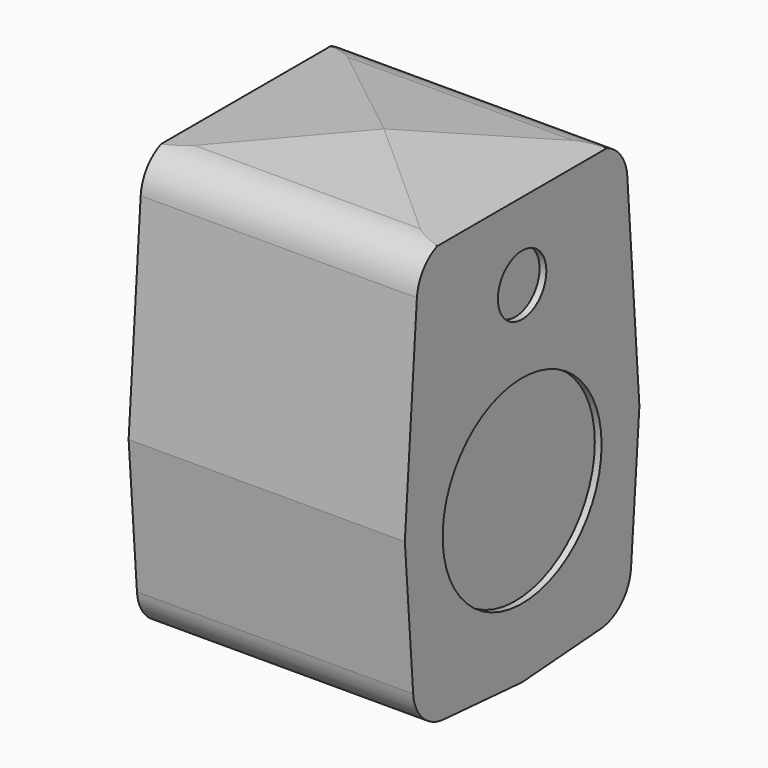
from build123d import *

# Parameters (mm, degrees)
F0_W         = 121
F0_H         = 195
F1_DEPTH     = 114
F3_DEPTH     = 114
F4_R         = 17
F6_DEPTH     = 134.1
F7_DEPTH     = 135.6
F2_R         = 41
F2_R_2       = 12.5
F8_DEPTH     = 2.8
F9_W         = 71.5012215078
F9_H         = 111.9857653975
F10_DEPTH    = 5
F11_W        = 35
F11_H        = 35
F12_DEPTH    = 35
F13_R        = 15
F14_DEPTH    = 35
F15_T1_DEPTH = 123.1187950266


# Not quite as in the source:
# - a fillet or chamfer that OpenCascade refuses, or shapes differently, is made with other operations: its cross-section is extruded or revolved along the edge and cut away or added


with BuildPart() as f1:
    # F0 (on Right) → F1 (new body)
    with BuildSketch(Plane.YZ):
        with Locations((-7.0141647011, 35.3717551942)):
            Rectangle(F0_W, F0_H)
    extrude(amount=F1_DEPTH)

    # F2 (on face) → F3 (cut, through all)
    with BuildSketch(Plane.YZ.offset(114)):
        Polygon((-60.2907269257, 126.0077205761), (-7.0141647011, 132.8717551942), (-67.5141647011, 132.8717551942), (-67.5141647011, 26.0932128876), align=None)
        Polygon((53.4858352989, 132.8717551942), (-7.0141647011, 132.8717551942), (46.2623975235, 126.0077205761), (53.4858352989, 26.0932128876), align=None)
        Polygon((-62.1019659576, -45.638720619), (-67.5141647011, 26.0932128876), (-67.5141647011, -62.1282448058), (53.4858352989, -62.1282448058), (53.4858352989, 26.0932128876), (48.0736365554, -45.638720619), (-7.0141647011, -49.6213585138), align=None)
    extrude(amount=-F3_DEPTH, mode=Mode.SUBTRACT)

    # F4
    f4_edges = [f1.edges().sort_by_distance(p)[0] for p in [
        (57, -60.290727, 126.007721),
        (57, 46.262398, 126.007721),
        (57, 48.073637, -45.638721),
        (57, -62.101966, -45.638721),
    ]]
    fillet(f4_edges, radius=F4_R)

    # F5 (on Front) → F6 (cut)
    with BuildSketch(Plane.XZ):
        Polygon((56.9999999998, 132.8717551942), (-2e-10, 132.8717551942), (-2e-10, 126.6480237246), align=None)
        Polygon((113.9999999999, 132.8717551942), (56.9999999998, 132.8717551942), (113.9999999999, 126.6480237246), align=None)
    extrude(amount=-F6_DEPTH, mode=Mode.SUBTRACT)

    # F5 (on Front) → F7 (cut)
    with BuildSketch(Plane.XZ):
        Polygon((56.9999999998, 132.8717551942), (-2e-10, 132.8717551942), (-2e-10, 126.6480237246), align=None)
        Polygon((113.9999999999, 132.8717551942), (56.9999999998, 132.8717551942), (113.9999999999, 126.6480237246), align=None)
    extrude(amount=F7_DEPTH, mode=Mode.SUBTRACT)

    # F2 (on face) → F8 (cut)
    with BuildSketch(Plane.YZ.offset(114)):
        with Locations((-7.0141647011, 19.9736393988)):
            Circle(F2_R)
        with Locations((-7.0141647011, 94.7317257524)):
            Circle(F2_R_2)
    extrude(amount=-F8_DEPTH, mode=Mode.SUBTRACT)

    # F9 (on face) → F10 (join)
    with BuildSketch(Plane(origin=(0, 0, 0), x_dir=(0, -1, 0), z_dir=(-1, 0, 0))):
        with Locations((7.0141647011, 18.3268077672)):
            Rectangle(F9_W, F9_H)
    extrude(amount=F10_DEPTH)

    # F11 (on face) → F12 (join)
    with BuildSketch(Plane(origin=(-5, 0, 0), x_dir=(0, -1, 0), z_dir=(-1, 0, 0))):
        with Locations((7.0141647011, 18.3268077672)):
            Rectangle(F11_W, F11_H)
    extrude(amount=F12_DEPTH)

    # F13 (on face) → F14 (cut, through all)
    with BuildSketch(Plane.XY.offset(35.8268077672)):
        with Locations((-22.5, -7.0141647011)):
            Circle(F13_R)
    extrude(amount=-F14_DEPTH, mode=Mode.SUBTRACT)

    # F15: fillet of radius 17.6237590053 on 2 edges, made by hand

    # F15_s2 → F15_t1 (cut)
    with BuildSketch(Plane.XY.offset(-43.2325897462)):
        with BuildLine():
            ThreePointArc((-22.3762409947, -24.5141647011), (-34.8381204973, -19.3522851984), (-40, -6.8904056958))
            Line((-40, -6.8904056958), (-40, -24.5141647011))
            Line((-40, -24.5141647011), (-22.3762409947, -24.5141647011))
        make_face()
        with BuildLine():
            ThreePointArc((-22.3762409947, 10.4858352989), (-34.8381204973, 5.3239557962), (-40, -7.1379237064))
            Line((-40, -7.1379237064), (-40, 10.4858352989))
            Line((-40, 10.4858352989), (-22.3762409947, 10.4858352989))
        make_face()
    extrude(amount=F15_T1_DEPTH, mode=Mode.SUBTRACT)


solid = f1.part
